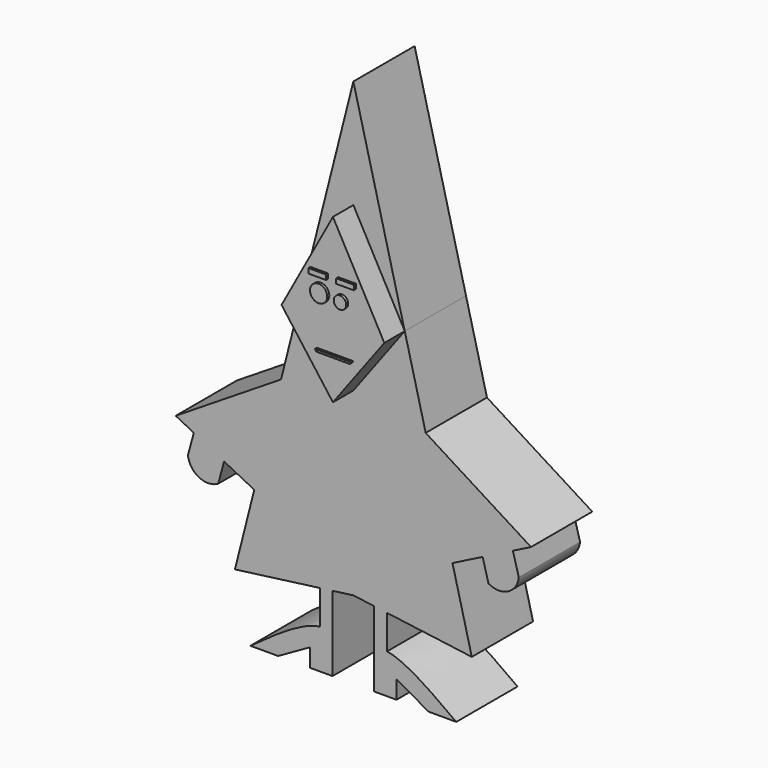
from build123d import *

# Parameters (mm, degrees)
F1_DEPTH = 19.05
F3_DEPTH = 6.35
F4_R     = 2.1395052033
F4_R_2   = 1.5473789097
F4_W     = 4.3834099779
F4_H     = 1.2019015849
F5_DEPTH = 0.635


with BuildPart() as f1:
    # F0 (on Front) → F1 (new body)
    with BuildSketch(Plane.XZ):
        Polygon((12.7812118899, 24.9824322697), (0, 75.4986554384), (-12.7812118899, 24.9824322697), (-17.9893098468, 4.3980431727), (17.9893098468, 4.3980431727), align=None)
        with BuildLine():
            Line((17.9893098468, 4.3980431727), (-17.9893098468, 4.3980431727))
            Line((-17.9893098468, 4.3980431727), (-44.1846288741, -12.0744779706))
            Line((-44.1846288741, -12.0744779706), (-39.6815885197, -14.3474328787))
            Line((-39.6815885197, -14.3474328787), (-41.1387868226, -19.7073649615))
            ThreePointArc((-41.1387868226, -19.7073649615), (-38.4139838362, -23.6659590485), (-33.6108808251, -23.5071512254))
            Line((-33.6108808251, -23.5071512254), (-32.1536825222, -18.1472191426))
            Line((-32.1536825222, -18.1472191426), (-24.6516230519, -21.933959112))
            Line((-24.6516230519, -21.933959112), (-29.4550578464, -40.9189650839))
            Line((-29.4550578464, -40.9189650839), (-8.3569039417, -38.1258840272))
            Line((-8.3569039417, -38.1258840272), (-8.3569039417, -46.5887725028))
            add(Edge.make_bspline(
                [(-8.3569039417, -46.5887725028), (-7.1639467181, -46.4381227358), (-6.0970060344, -46.567074298), (-5.1892242436, -47.0491623459)],
                knots=[0.3623606656, 0.3623606656, 0.3623606656, 0.3623606656, 0.4576615295, 0.4576615295, 0.4576615295, 0.4576615295], degree=3))
            Line((-5.1892242436, -47.0491623459), (-5.1892242436, -37.7065304572))
            Line((-5.1892242436, -37.7065304572), (0, -37.0195545256))
            Line((0, -37.0195545256), (5.1886305738, -37.7110000757))
            Line((5.1886305738, -37.7110000757), (5.1805830548, -47.0536284984))
            add(Edge.make_bspline(
                [(8.3486581466, -46.5959673895), (7.1558311316, -46.4442900935), (6.0887797679, -46.5723225708), (5.1805830548, -47.0536284984)],
                knots=[0.3623606656, 0.3623606656, 0.3623606656, 0.3623606656, 0.4576615295, 0.4576615295, 0.4576615295, 0.4576615295], degree=3))
            Line((8.3486581466, -46.5959673895), (8.3559478758, -38.1330820534))
            Line((8.3559478758, -38.1330820534), (29.4550578464, -40.9189650839))
            Line((29.4550578464, -40.9189650839), (24.6516230519, -21.933959112))
            Line((24.6516230519, -21.933959112), (32.1536825222, -18.1472191426))
            Line((32.1536825222, -18.1472191426), (33.6108808251, -23.5071512254))
            ThreePointArc((33.6108808251, -23.5071512254), (38.4139838362, -23.6659590485), (41.1387868226, -19.7073649615))
            Line((41.1387868226, -19.7073649615), (39.6815885197, -14.3474328787))
            Line((39.6815885197, -14.3474328787), (44.1846288741, -12.0744779706))
            Line((44.1846288741, -12.0744779706), (17.9893098468, 4.3980431727))
        make_face()
        with BuildLine():
            add(Edge.make_bspline(
                [(-8.3569039417, -46.5887725028), (-7.1639467181, -46.4381227358), (-6.0970060344, -46.567074298), (-5.1892242436, -47.0491623459)],
                knots=[0.3623606656, 0.3623606656, 0.3623606656, 0.3623606656, 0.4576615295, 0.4576615295, 0.4576615295, 0.4576615295], degree=3))
            add(Edge.make_bspline(
                [(-25.6085079163, -56.3917942345), (-19.2506852316, -51.7766897434), (-12.8928625468, -47.1615852522), (-8.3569039417, -46.5887725028)],
                knots=[0, 0, 0, 0, 0.3623606656, 0.3623606656, 0.3623606656, 0.3623606656], degree=3))
            Line((-25.6085079163, -56.3917942345), (-18.7088064849, -56.3917942345))
            Line((-18.7088064849, -56.3917942345), (-10.747612454, -51.8804490566))
            Line((-10.747612454, -51.8804490566), (-10.747612454, -56.3917942345))
            Line((-10.747612454, -56.3917942345), (-5.1892242436, -56.3917942345))
            Line((-5.1892242436, -56.3917942345), (-5.1892242436, -47.0491623459))
        make_face()
        with BuildLine():
            add(Edge.make_bspline(
                [(25.5918116332, -56.4138456024), (19.2379666475, -51.7932663474), (12.8841216618, -47.1726870923), (8.3486581466, -46.5959673895)],
                knots=[0, 0, 0, 0, 0.3623606656, 0.3623606656, 0.3623606656, 0.3623606656], degree=3))
            add(Edge.make_bspline(
                [(8.3486581466, -46.5959673895), (7.1558311316, -46.4442900935), (6.0887797679, -46.5723225708), (5.1805830548, -47.0536284984)],
                knots=[0.3623606656, 0.3623606656, 0.3623606656, 0.3623606656, 0.4576615295, 0.4576615295, 0.4576615295, 0.4576615295], degree=3))
            Line((5.1805830548, -47.0536284984), (5.1725355357, -56.396256921))
            Line((5.1725355357, -56.396256921), (10.730921684, -56.4010447834))
            Line((10.730921684, -56.4010447834), (10.7348076486, -51.8897012791))
            Line((10.7348076486, -51.8897012791), (18.6921127615, -56.407902365))
            Line((18.6921127615, -56.407902365), (25.5918116332, -56.4138456024))
        make_face()
    extrude(amount=F1_DEPTH)

    # F2 (on face) → F3 (join)
    with BuildSketch(Plane.XZ.offset(19.05)):
        Polygon((12.7791271915, 24.9906717928), (0, 48.4305992723), (-12.7791271915, 24.9906717928), (0, 7.8285075724), align=None)
    extrude(amount=F3_DEPTH)

    # F4 (on face) → F5 (join)
    with BuildSketch(Plane.XZ.offset(25.4)):
        with Locations((-3.0517904088, 30.9159699827)):
            Circle(F4_R)
        with Locations((2.2556707263, 30.6505970657)):
            Circle(F4_R_2)
        Polygon((5.0654464612, 18.4789821506), (-3.9945594035, 18.4789821506), (-3.6306733055, 17.9902889184), (4.7015603632, 17.9902889184), align=None)
        with Locations((-3.4289575997, 35.0581686944)):
            Rectangle(F4_W, F4_H)
        with Locations((3.4996584873, 35.0581686944)):
            Rectangle(F4_W, F4_H)
    extrude(amount=F5_DEPTH)


solid = f1.part
